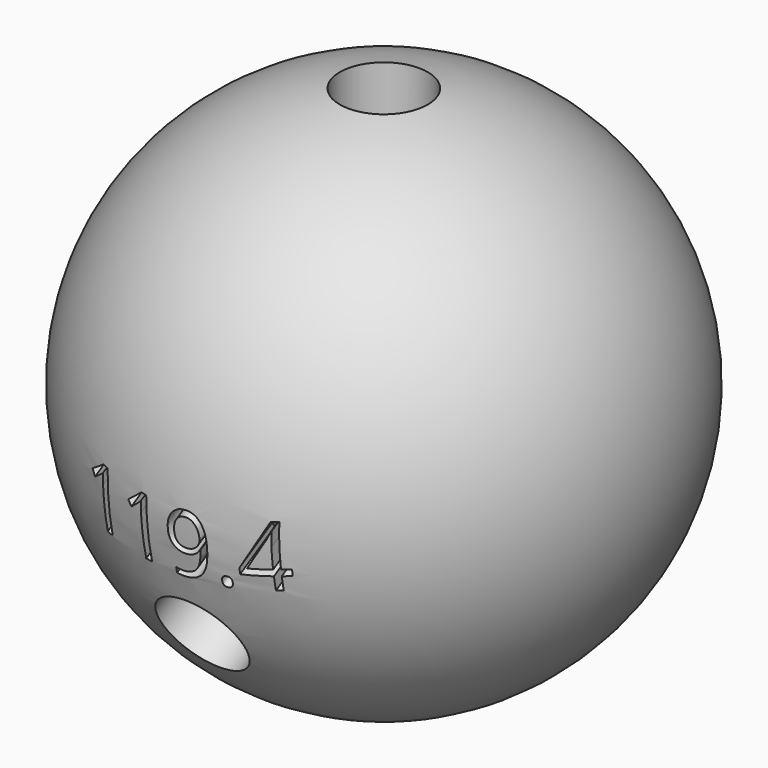
from build123d import *

# Parameters (mm, degrees)
F5_R          = 3.175
F6_DEPTH      = 76.2
F7_ANGLE      = 119.4
F8_ANGLE      = 124.6
F10_TEXT_SIZE = 5.7784387738
F11_DEPTH     = 6.35
F13_TEXT_SIZE = 6.645384969
F14_DEPTH     = 6.35


# Not quite as in the source:
# - Text() gives the source's letters only with a copy of the font that has no kerning and outlines rounded to 1/6400 em; it was checked with that copy


with BuildPart() as f2:
    # F0 (on Front) → F2 (revolve)
    with BuildSketch(Plane.XZ):
        with BuildLine():
            Line((0, -19.05), (0, 19.05))
            ThreePointArc((0, 19.05), (-19.05, 0), (0, -19.05))
        make_face()
    revolve(axis=Axis((0, 0, 0), (0, 0, 1)))

    # F10 (on offset) → F11 (cut)
    with BuildSketch(Plane(origin=(0, -17.703064642, -9.9751642735), x_dir=(1, 0, 0), z_dir=(0, -0.8712138111, -0.4909037536))):
        with Locations((-7.3158596642, 5.1700836048)):
            Text('119.4', F10_TEXT_SIZE, font='Open Sans', text_align=(TextAlign.LEFT, TextAlign.BOTTOM))
    extrude(amount=-F11_DEPTH, mode=Mode.SUBTRACT)

    # F13 (on offset) → F14 (cut)
    with BuildSketch(Plane(origin=(0, 18.2634950208, -8.9077017028), x_dir=(-1, 0, 0), z_dir=(0, 0.8987940463, -0.4383711468))):
        with Locations((-8.5362046609, 4.848905839)):
            Text('124.6', F13_TEXT_SIZE, font='Open Sans', text_align=(TextAlign.LEFT, TextAlign.BOTTOM))
    extrude(amount=-F14_DEPTH, mode=Mode.SUBTRACT)


with BuildPart() as f6:
    # F5 (on offset) → F6 (new body)
    with BuildSketch(Plane.XY.offset(7.62)):
        Circle(F5_R)
    extrude(amount=F6_DEPTH)


with BuildPart() as f7_1:
    # F7: copy of F6
    add(f6.part.rotate(Axis((38.1614528596, 0, 0), (1, 0, 0)), F7_ANGLE))


with BuildPart() as f8_1:
    # F8: copy of F7_1
    add(f7_1.part.rotate(Axis((38.1614528596, 0, 0), (1, 0, 0)), F8_ANGLE))


with BuildPart() as f2_1:
    add(f2.part)

    # F15: cut F6, F8_1, F7_1
    add(f6.part, mode=Mode.SUBTRACT)
    add(f8_1.part, mode=Mode.SUBTRACT)
    add(f7_1.part, mode=Mode.SUBTRACT)


solid = f2_1.part
